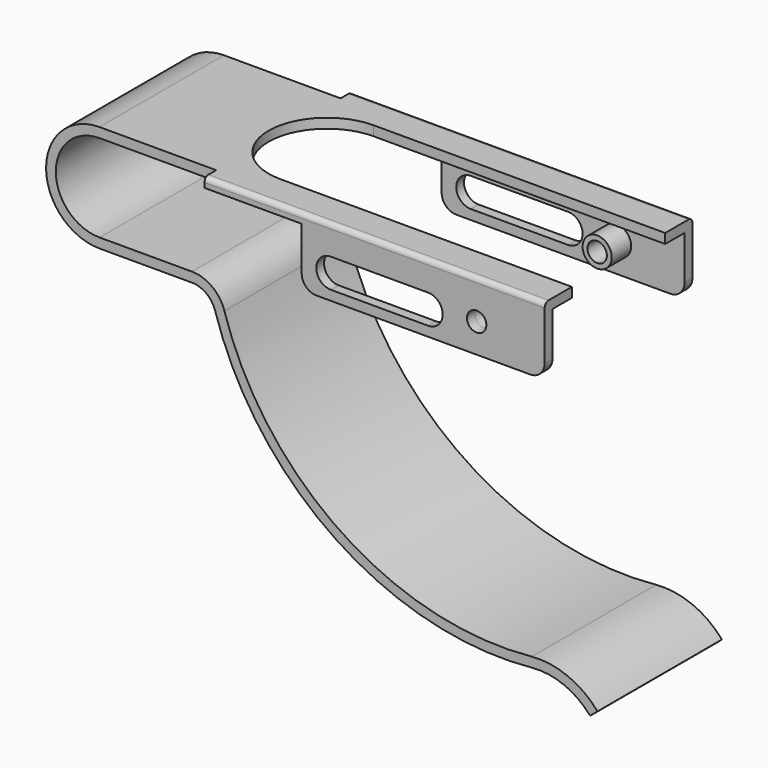
from build123d import *

# Parameters (mm, degrees)
F1_DEPTH  = 16
F2_W      = 70
F2_H      = 3
F3_DEPTH  = 2
F4_W      = 50
F4_H      = 14
F5_DEPTH  = 2
F6_R      = 1
F9_DEPTH  = 32.3
F11_DEPTH = 38.001
F13_D     = 4
F14_R     = 3
F14_R_2   = 2
F15_DEPTH = 5
F16_R     = 3


# Not quite as in the source:
# - ends of sketch curves that miss each other by under 0.0002 mm in the source are joined
# - a pattern or mirror of a feature is missing from the dataset's text; its kind, count and spacing are read off the source's solid


with BuildPart() as f1:
    # F0 (on Front) → F1 (new body)
    with BuildSketch(Plane.XZ):
        with BuildLine():
            Line((94, 10.9999997337), (0, 10.9999997337))
            ThreePointArc((0, 10.9999997337), (-10.9999997337, 0), (0, -10.9999997337))
            Line((0, -10.9999997337), (19, -10.9999997337))
            ThreePointArc((19, -10.9999997337), (21.9703860558, -11.9779596195), (23.7788047483, -14.5292770618))
            ThreePointArc((23.7788047483, -14.5292770618), (48.7042113744, -47.9191442908), (89.135710582, -57.9915323328))
            ThreePointArc((89.135710582, -57.9915323328), (95.6273356348, -58.9810862831), (100.9536755577, -62.8217263174))
            Line((100.9536755577, -62.8217263174), (102.4712510554, -61.5190536469))
            ThreePointArc((102.4712510554, -61.5190536469), (96.3776978188, -57.1271725396), (88.9514269277, -56))
            ThreePointArc((88.9514269277, -56), (49.8169100213, -46.2572353593), (25.6903263931, -13.9409880714))
            ThreePointArc((25.6903263931, -13.9409880714), (23.1585403199, -10.3691437881), (19, -9))
            Line((19, -9), (0, -9))
            ThreePointArc((0, -9), (-9, 0), (0, 9))
            Line((0, 9), (94, 9))
            Line((94, 9), (94, 10.9999997337))
        make_face()
    extrude(amount=F1_DEPTH)

    # F2 (on face) → F3 (join)
    with BuildSketch(Plane.XY.offset(10.9999997337)):
        with Locations((59, -17.5)):
            Rectangle(F2_W, F2_H)
    extrude(amount=-F3_DEPTH)

    # F4 (on face) → F5 (join)
    with BuildSketch(Plane.XZ.offset(19)):
        with Locations((69, 3.9999997337)):
            Rectangle(F4_W, F4_H)
    extrude(amount=-F5_DEPTH)

    # F6
    f6_edges = [f1.edges().sort_by_distance(p)[0] for p in [
        (59, -19, 11),
    ]]
    fillet(f6_edges, radius=F6_R)

    # F7: F1 across plane


with BuildPart() as f1_1:
    add(f1.part)
    add(f1.part.mirror(Plane.XZ))

    # F8 (on Top) → F9 (cut)
    with BuildSketch(Plane.XY):
        with BuildLine():
            Line((94, 12), (34, 12))
            ThreePointArc((34, 12), (22, 0), (34, -12))
            Line((34, -12), (94, -12))
            Line((94, -12), (94, 12))
        make_face()
    extrude(amount=F9_DEPTH, mode=Mode.SUBTRACT)

    # F10 (on face) → F11 (cut, through all)
    with BuildSketch(Plane.XZ.offset(19)):
        with BuildLine():
            ThreePointArc((50, 4.9999997337), (47, 1.9999997337), (50, -1.0000002663))
            Line((50, -1.0000002663), (70, -1.0000002663))
            ThreePointArc((70, -1.0000002663), (73, 1.9999997337), (70, 4.9999997337))
            Line((70, 4.9999997337), (50, 4.9999997337))
        make_face()
    extrude(amount=-F11_DEPTH, mode=Mode.SUBTRACT)

    # F13 (through all)
    with Locations(Plane.XZ.offset(19)):
        with Locations((80, 2.9999997337)):
            Hole(F13_D / 2)

    # F14 (on face) → F15 (join)
    with BuildSketch(Plane(origin=(0, -17, 0), x_dir=(-1, 0, 0), z_dir=(0, 1, 0))):
        with Locations((-80, 2.9999997337)):
            Circle(F14_R)
        with Locations((-80, 2.9999997337)):
            Circle(F14_R_2, mode=Mode.SUBTRACT)
    f15 = extrude(amount=F15_DEPTH)

    # F15_copies: F15 across plane
    add(f15.mirror(Plane.ZX))

    # F16
    f16_edges = [f1_1.edges().sort_by_distance(p)[0] for p in [
        (94, -18, -3),
        (94, 18, -3),
        (44, -18, -3),
        (44, 18, -3),
    ]]
    fillet(f16_edges, radius=F16_R)


solid = f1_1.part
